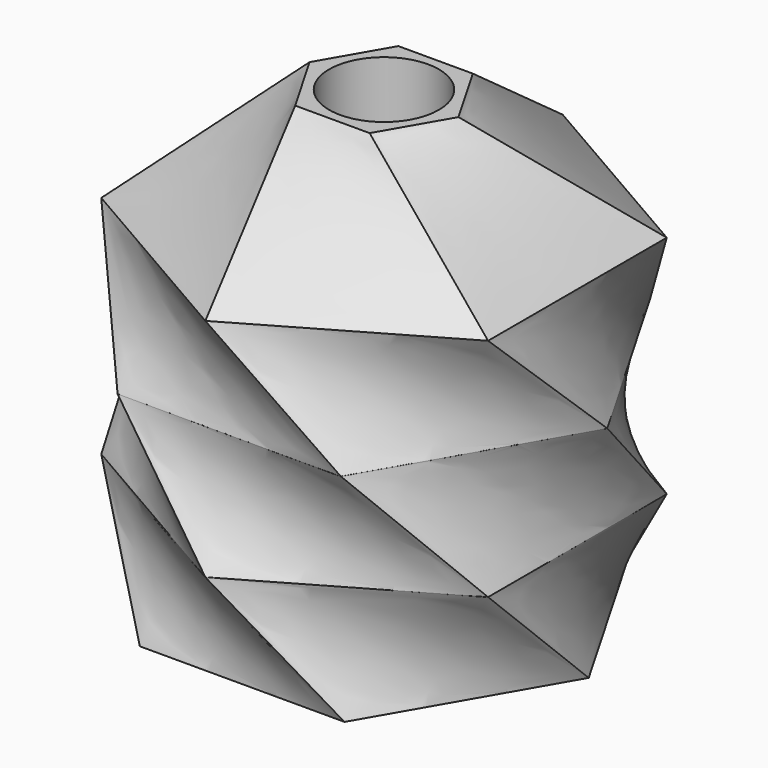
from build123d import *

# Parameters (mm, degrees)
F13_R     = 17.029051
F14_DEPTH = 140.001
F15_R     = 52.162702
F16_DEPTH = 30


with BuildPart() as f9:
    # F4 (on Top) → F9 section 0
    with BuildSketch(Plane.XY):
        Polygon((-31.754265, -55), (31.754265, -55), (63.50853, 0), (31.754265, 55), (-31.754265, 55), (-63.50853, 0), align=None)
    # F5 (on offset) → F9 section 1
    with BuildSketch(Plane.XY.offset(35)):
        Polygon((60, -34.641016), (60, 34.641016), (0, 69.282032), (-60, 34.641016), (-60, -34.641016), (0, -69.282032), align=None)
    loft()

    # F5 (on offset) → F10 section 0
    with BuildSketch(Plane.XY.offset(35)):
        Polygon((60, -34.641016), (60, 34.641016), (0, 69.282032), (-60, 34.641016), (-60, -34.641016), (0, -69.282032), align=None)
    # F6 (on offset) → F10 section 1
    with BuildSketch(Plane.XY.offset(70)):
        Polygon((34.641016, -60), (69.282032, 0), (34.641016, 60), (-34.641016, 60), (-69.282032, 0), (-34.641016, -60), align=None)
    loft()

    # F6 (on offset) → F11 section 0
    with BuildSketch(Plane.XY.offset(70)):
        Polygon((34.641016, -60), (69.282032, 0), (34.641016, 60), (-34.641016, 60), (-69.282032, 0), (-34.641016, -60), align=None)
    # F7 (on offset) → F11 section 1
    with BuildSketch(Plane.XY.offset(105)):
        Polygon((0, -69.282032), (60, -34.641016), (60, 34.641016), (0, 69.282032), (-60, 34.641016), (-60, -34.641016), align=None)
    loft()

    # F7 (on offset) → F12 section 0
    with BuildSketch(Plane.XY.offset(105)):
        Polygon((0, -69.282032), (60, -34.641016), (60, 34.641016), (0, 69.282032), (-60, 34.641016), (-60, -34.641016), align=None)
    # F8 (on offset) → F12 section 1
    with BuildSketch(Plane.XY.offset(140)):
        Polygon((11.547005, -20), (23.094011, 0), (11.547005, 20), (-11.547005, 20), (-23.094011, 0), (-11.547005, -20), align=None)
    loft()

    # F13 (on face) → F14 (cut, through all)
    with BuildSketch(Plane.XY.offset(140)):
        Circle(F13_R)
    extrude(amount=-F14_DEPTH, mode=Mode.SUBTRACT)

    # F15 (on face) → F16 (cut)
    with BuildSketch(Plane.XY):
        Circle(F15_R)
    extrude(amount=F16_DEPTH, mode=Mode.SUBTRACT)


solid = f9.part
